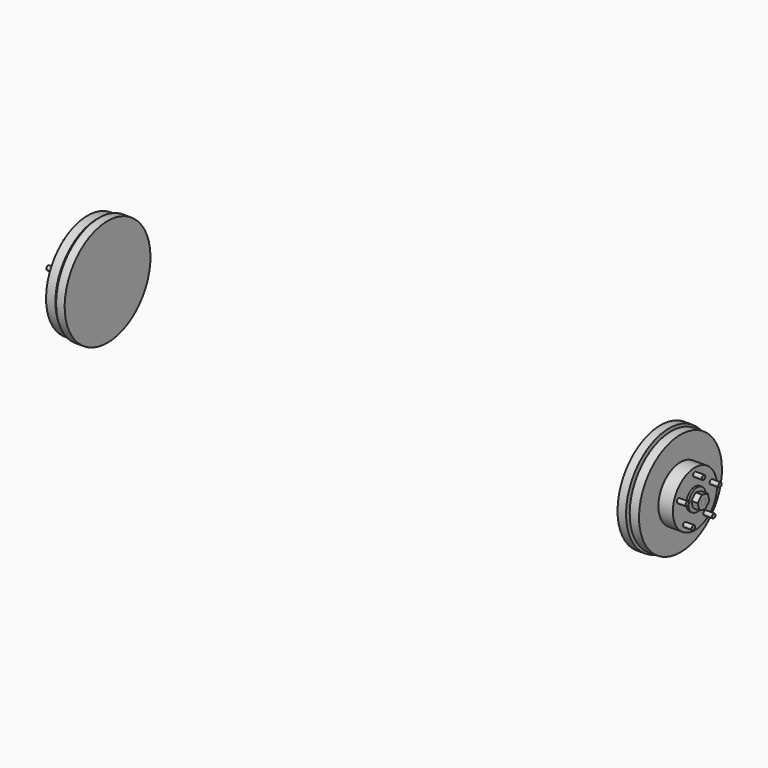
from build123d import *

# Parameters (mm, degrees)
F6_R      = 6.35
F7_DEPTH  = 25.4
F8_R      = 31.75
F8_R_2    = 10.31875
F9_DEPTH  = 6.35
F10_R     = 8.7376
F11_DEPTH = 19.05


# Not quite as in the source:
# - a feature of the source that left no trace in its solid (it failed there, or was rolled back) is left out


with BuildPart() as f2:
    # F1 (on Front) → F2 (revolve)
    with BuildSketch(Plane.XZ):
        Polygon((895.35, -9.525), (914.4, -9.525), (939.8, -9.525), (939.8, 0), (812.9769563675, 0), (812.9769563675, -157.7237546444), (838.0940758705, -157.7237546444), (838.0940758705, -18.3208048281), (841.2690758705, -18.3208048281), (841.2690758705, -11.9708048281), (844.4440758705, -11.8136759589), (869.8440758705, -10.5566450056), (890.6898498535, -9.525), align=None)
    revolve(axis=Axis((876.3884781837, 0, 0), (-1, 0, 0)))


with BuildPart() as f3:
    # F1 (on Front) → F3 (revolve)
    with BuildSketch(Plane.XZ):
        Polygon((914.4, -81.2187399507), (914.4, -25.4), (895.35, -25.4), (895.35, -12.065), (879.4372081757, -12.065), (869.8440758705, -12.2509578667), (869.8440758705, -38.1), (844.4440758705, -38.1), (844.4440758705, -152.4), (871.9114001578, -152.4), (871.9114001578, -81.2187399507), align=None)
    revolve(axis=Axis((876.3884781837, 0, 0), (-1, 0, 0)))

    # F6 (on face) → F7 (join)
    with BuildSketch(Plane.YZ.offset(914.4)):
        with Locations((0, 63.5)):
            Circle(F6_R)
        with Locations((-60.3920887847, 19.6225791428)):
            Circle(F6_R)
        with Locations((-37.3243635206, -51.3725791428)):
            Circle(F6_R)
        with Locations((37.3243635206, -51.3725791428)):
            Circle(F6_R)
        with Locations((60.3920887847, 19.6225791428)):
            Circle(F6_R)
    extrude(amount=F7_DEPTH)


with BuildPart() as f4:
    # F1 (on Front) → F4 (revolve)
    with BuildSketch(Plane.XZ):
        Polygon((869.8440758705, -38.1), (869.8440758705, -12.2509578667), (869.8440758705, -10.5566450056), (844.4440758705, -11.8136759589), (844.4440758705, -38.1), align=None)
    revolve(axis=Axis((876.3884781837, 0, 0), (-1, 0, 0)))


with BuildPart() as f5:
    # F1 (on Front) → F5 (revolve)
    with BuildSketch(Plane.XZ):
        Polygon((895.35, -25.4), (914.4, -25.4), (914.4, -9.525), (895.35, -9.525), (895.35, -12.065), align=None)
    revolve(axis=Axis((876.3884781837, 0, 0), (-1, 0, 0)))


with BuildPart() as f9:
    # F8 (on face) → F9 (new body)
    with BuildSketch(Plane.YZ.offset(914.4)):
        Circle(F8_R)
        Circle(F8_R_2, mode=Mode.SUBTRACT)
    extrude(amount=F9_DEPTH)


with BuildPart() as f11:
    # F10 (on face) → F11 (new body)
    with BuildSketch(Plane.YZ.offset(920.75)):
        Polygon((15.4993414366, 15.6089850737), (-5.7681068828, 21.2273159629), (-21.2674483194, 5.6183308892), (-15.4993414366, -15.6089850737), (5.7681068828, -21.2273159629), (21.2674483194, -5.6183308892), align=None)
        Circle(F10_R, mode=Mode.SUBTRACT)
    extrude(amount=F11_DEPTH)


with BuildPart() as f12_1:
    # F12: instance of F2
    add(f2.part.mirror(Plane.YZ))


with BuildPart() as f12_2:
    # F12: instance of F3
    add(f3.part.mirror(Plane.YZ))


with BuildPart() as f12_3:
    # F12: instance of F4
    add(f4.part.mirror(Plane.YZ))


with BuildPart() as f12_4:
    # F12: instance of F5
    add(f5.part.mirror(Plane.YZ))


with BuildPart() as f12_5:
    # F12: instance of F9
    add(f9.part.mirror(Plane.YZ))


with BuildPart() as f12_6:
    # F12: instance of F11
    add(f11.part.mirror(Plane.YZ))


solid = Compound([f2.part, f3.part, f4.part, f5.part, f9.part, f11.part, f12_1.part, f12_2.part, f12_3.part, f12_4.part, f12_5.part, f12_6.part])
